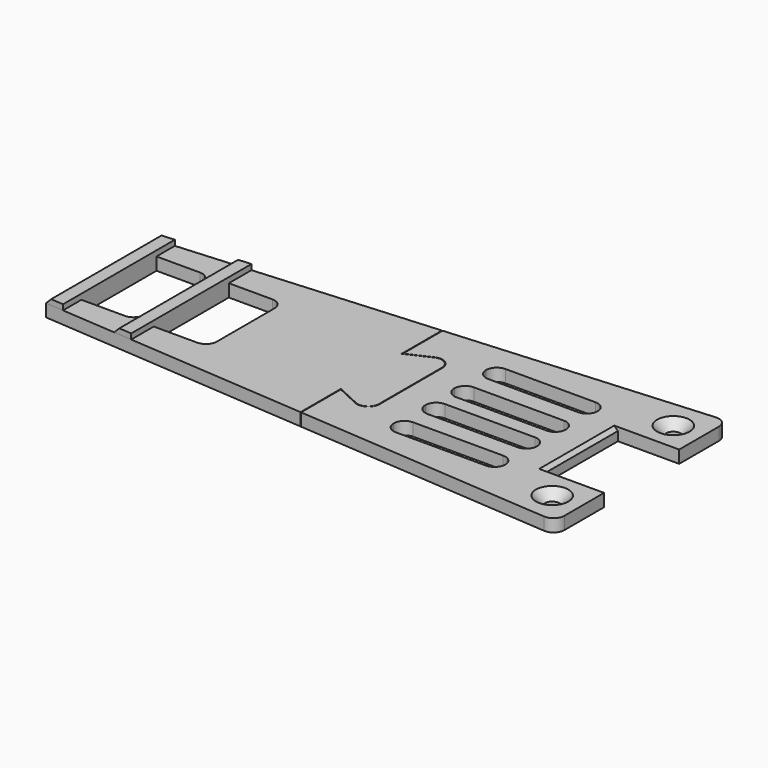
from build123d import *

# Parameters (mm, degrees)
F0_W     = 15.0803372804
F0_H     = 26.0359900557
F1_DEPTH = 3.5
F0_W_2   = 30.9743065556
F0_H_2   = 6
F0_R     = 2
F2_SIZE  = 1
F3_SIZE  = 2.5
F5_DEPTH = 1.5
F6_R     = 3
F7_SIZE  = 1.49999
F8_R     = 3
F9_R     = 2.99999


# Not quite as in the source:
# - a fillet or chamfer is up to 0.001 mm smaller than in the source, because OpenCascade refuses the exact size


with BuildPart() as f1:
    # F0 (on Top) → F1 (new body)
    with BuildSketch(Plane.XY):
        with BuildLine():
            Line((5.6491911411, 26.5359900557), (-69.3508088589, 21.0359900557))
            Line((-69.3508088589, 21.0359900557), (-69.3508088589, -17))
            Line((-69.3508088589, -17), (5.6491911411, -22.5))
            Line((5.6491911411, -22.5), (5.6491911411, -8.5))
            Line((5.6491911411, -8.5), (12.2570298003, -11.5812857706))
            ThreePointArc((12.2570298003, -11.5812857706), (15.1367834106, -11.392536747), (16.5248845856, -8.8623624095))
            Line((16.5248845856, -8.8623624095), (16.5248845856, 12.8983524652))
            ThreePointArc((16.5248845856, 12.8983524652), (15.1367834106, 15.4285268026), (12.2570298003, 15.6172758263))
            Line((12.2570298003, 15.6172758263), (5.6491911411, 12.5359900557))
            Line((5.6491911411, 12.5359900557), (5.6491911411, 26.5359900557))
        make_face()
        with Locations((-56.8106402187, 2.0179950278)):
            Rectangle(F0_W, F0_H, mode=Mode.SUBTRACT)
        with Locations((-36.7303029383, 2.0000000728)):
            Rectangle(F0_W, F0_H, mode=Mode.SUBTRACT)
    extrude(amount=F1_DEPTH)

    # F4 (on face) → F5 (join)
    with BuildSketch(Plane.XY.offset(3.5)):
        Polygon((-64.3508088589, 21.4026567223), (-69.3508088589, 21.0359900557), (-69.3508088589, -17), (-64.3508088589, -17.3666666667), (-64.3508088589, -11), (-64.3508088589, 15.0359900557), align=None)
        Polygon((-44.2704715785, 22.8752147895), (-49.2704715785, 22.5085481229), (-49.2704715785, 15.0359900557), (-49.2704715785, -11), (-49.2704715785, -18.4725580672), (-44.2704715785, -18.8392247339), (-44.2704715785, -11.0179949551), (-44.2704715785, 15.0179951006), align=None)
    extrude(amount=F5_DEPTH)

    # F6
    f6_edges = [f1.edges().sort_by_distance(p)[0] for p in [
        (-49.270472, 15.03599, 1.75),
        (-29.190134, 15.017995, 1.75),
        (-49.270472, -11, 1.75),
        (-29.190134, -11.017995, 1.75),
    ]]
    fillet(f6_edges, radius=F6_R)

    # F7 (size 1.5 in the source; OpenCascade refuses exactly that, so slightly less here)
    f7_edges = [f1.edges().sort_by_distance(p)[0] for p in [
        (-69.350809, 2.017995, 5),
        (-49.270472, 2.017995, 5),
    ]]
    chamfer(f7_edges, length=F7_SIZE)


with BuildPart() as f1b:
    # F0 (on Top) → F1, piece 2 (new body)
    with BuildSketch(Plane.XY):
        with BuildLine():
            Line((5.7991911411, -22.511), (80.6491911411, -28))
            Line((80.6491911411, -28), (80.6491911411, -11))
            Line((80.6491911411, -11), (63.6491911411, -11))
            Line((63.6491911411, -11), (63.6491911411, 15.0359900557))
            Line((63.6491911411, 15.0359900557), (80.6491911411, 15.0359900557))
            Line((80.6491911411, 15.0359900557), (80.6491911411, 32.0359900557))
            Line((80.6491911411, 32.0359900557), (5.7991911411, 26.5469900557))
            Line((5.7991911411, 26.5469900557), (5.7991911411, 12.7714428922))
            Line((5.7991911411, 12.7714428922), (12.1936370611, 15.7532219944))
            ThreePointArc((12.1936370611, 15.7532219944), (15.2173783519, 15.5550355195), (16.6748845856, 12.8983524652))
            Line((16.6748845856, 12.8983524652), (16.6748845856, -8.8623624095))
            ThreePointArc((16.6748845856, -8.8623624095), (15.2173783519, -11.5190454638), (12.1936370611, -11.7172319387))
            Line((12.1936370611, -11.7172319387), (5.7991911411, -8.7354528366))
            Line((5.7991911411, -8.7354528366), (5.7991911411, -22.511))
        make_face()
        with Locations((40.1620378633, -14)):
            Rectangle(F0_W_2, F0_H_2, mode=Mode.SUBTRACT)
        with Locations((72.6491911411, -19)):
            Circle(F0_R, mode=Mode.SUBTRACT)
        with Locations((40.1620378633, -3)):
            Rectangle(F0_W_2, F0_H_2, mode=Mode.SUBTRACT)
        with Locations((40.1620378633, 7.0359900557)):
            Rectangle(F0_W_2, F0_H_2, mode=Mode.SUBTRACT)
        with Locations((40.1620378633, 18.0359900557)):
            Rectangle(F0_W_2, F0_H_2, mode=Mode.SUBTRACT)
        with Locations((72.6491911411, 23)):
            Circle(F0_R, mode=Mode.SUBTRACT)
    extrude(amount=F1_DEPTH)

    # F2
    f2_edges = [f1b.edges().sort_by_distance(p)[0] for p in [
        (63.649191, 2.017995, 3.5),
    ]]
    chamfer(f2_edges, length=F2_SIZE)

    # F3
    f3_edges = [f1b.edges().sort_by_distance(p)[0] for p in [
        (70.649191, 23, 3.5),
        (70.649191, -19, 3.5),
    ]]
    chamfer(f3_edges, length=F3_SIZE)

    # F8
    f8_edges = [f1b.edges().sort_by_distance(p)[0] for p in [
        (80.649191, 32.03599, 1.75),
        (80.649191, -28, 1.75),
    ]]
    fillet(f8_edges, radius=F8_R)

    # F9 (radius 3 in the source; OpenCascade refuses exactly that, so slightly less here)
    f9_edges = [f1b.edges().sort_by_distance(p)[0] for p in [
        (24.674885, 21.03599, 1.75),
        (24.674885, 10.03599, 1.75),
        (24.674885, 0, 1.75),
        (24.674885, -11, 1.75),
        (24.674885, 15.03599, 1.75),
        (24.674885, 4.03599, 1.75),
        (24.674885, -6, 1.75),
        (24.674885, -17, 1.75),
        (55.649191, 21.03599, 1.75),
        (55.649191, 10.03599, 1.75),
        (55.649191, 0, 1.75),
        (55.649191, -11, 1.75),
        (55.649191, -17, 1.75),
        (55.649191, -6, 1.75),
        (55.649191, 4.03599, 1.75),
        (55.649191, 15.03599, 1.75),
    ]]
    fillet(f9_edges, radius=F9_R)


solid = Compound([f1.part, f1b.part])
